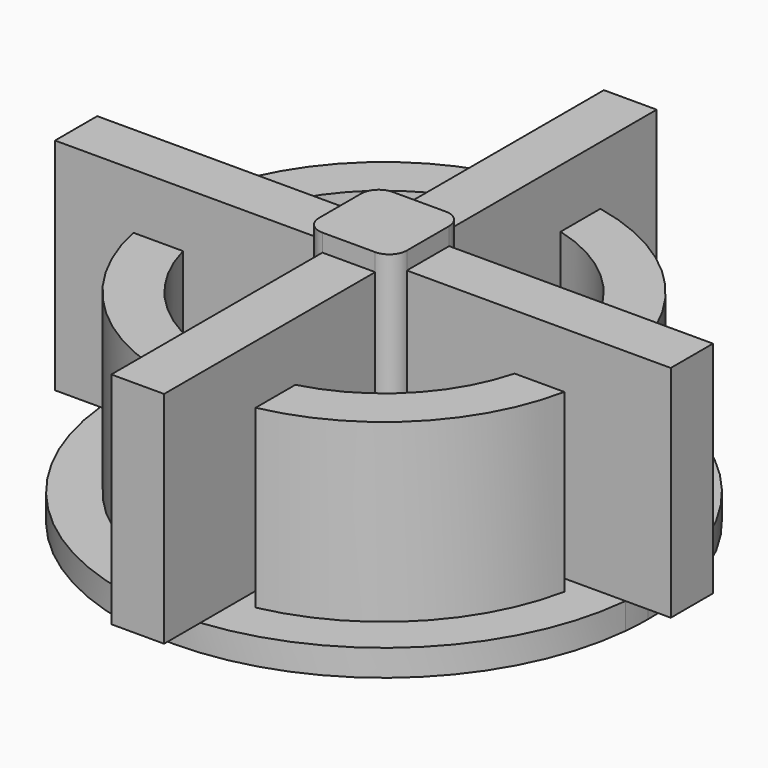
from build123d import *

# Parameters (mm, degrees)
F1_DEPTH = 3
F2_DEPTH = 20
F3_DEPTH = 25
F4_DEPTH = 27


with BuildPart() as f1:
    # F0 (on Top) → F1 (new body)
    with BuildSketch(Plane.XY):
        with BuildLine():
            Line((29.8496231132, -3), (24.819347292, -3))
            ThreePointArc((24.819347292, -3), (24.6773921449, -4.0032882645), (24.4948974278, -5))
            ThreePointArc((24.4948974278, -5), (17.6776695297, -17.6776695297), (5, -24.4948974278))
            ThreePointArc((5, -24.4948974278), (4.0032882645, -24.6773921449), (3, -24.819347292))
            Line((3, -24.819347292), (3, -29.8496231132))
            ThreePointArc((3, -29.8496231132), (21.2132034356, -21.2132034356), (29.8496231132, -3))
        make_face()
        with BuildLine():
            ThreePointArc((5, -24.4948974278), (17.6776695297, -17.6776695297), (24.4948974278, -5))
            Line((24.4948974278, -5), (18.848076825, -5))
            ThreePointArc((18.848076825, -5), (13.7885822331, -13.7885822331), (5, -18.848076825))
            Line((5, -18.848076825), (5, -24.4948974278))
        make_face()
        with BuildLine():
            ThreePointArc((24.4948974278, -5), (24.6773921449, -4.0032882645), (24.819347292, -3))
            Line((24.819347292, -3), (19.267848868, -3))
            ThreePointArc((19.267848868, -3), (19.0841805655, -4.0055027327), (18.848076825, -5))
            Line((18.848076825, -5), (24.4948974278, -5))
        make_face()
        with BuildLine():
            ThreePointArc((25, 0), (24.9547959549, 1.5027171558), (24.819347292, 3))
            Line((24.819347292, 3), (19.267848868, 3))
            ThreePointArc((19.267848868, 3), (19.4418755902, 1.5044844755), (19.5, 0))
            ThreePointArc((19.5, 0), (19.4418755902, -1.5044844755), (19.267848868, -3))
            Line((19.267848868, -3), (24.819347292, -3))
            ThreePointArc((24.819347292, -3), (24.9547959549, -1.5027171558), (25, 0))
        make_face()
        with BuildLine():
            ThreePointArc((24.819347292, 3), (24.6773921449, 4.0032882645), (24.4948974278, 5))
            Line((24.4948974278, 5), (18.848076825, 5))
            ThreePointArc((18.848076825, 5), (19.0841805655, 4.0055027327), (19.267848868, 3))
            Line((19.267848868, 3), (24.819347292, 3))
        make_face()
        with BuildLine():
            Line((18.848076825, 5), (24.4948974278, 5))
            ThreePointArc((24.4948974278, 5), (17.6776695297, 17.6776695297), (5, 24.4948974278))
            Line((5, 24.4948974278), (5, 18.848076825))
            ThreePointArc((5, 18.848076825), (13.7885822331, 13.7885822331), (18.848076825, 5))
        make_face()
        with BuildLine():
            ThreePointArc((5, 24.4948974278), (17.6776695297, 17.6776695297), (24.4948974278, 5))
            ThreePointArc((24.4948974278, 5), (24.6773921449, 4.0032882645), (24.819347292, 3))
            Line((24.819347292, 3), (29.8496231132, 3))
            ThreePointArc((29.8496231132, 3), (21.2132034356, 21.2132034356), (3, 29.8496231132))
            Line((3, 29.8496231132), (3, 24.819347292))
            ThreePointArc((3, 24.819347292), (4.0032882645, 24.6773921449), (5, 24.4948974278))
        make_face()
        with BuildLine():
            Line((29.8496231132, 3), (24.819347292, 3))
            ThreePointArc((24.819347292, 3), (24.9547959549, 1.5027171558), (25, 0))
            ThreePointArc((25, 0), (24.9547959549, -1.5027171558), (24.819347292, -3))
            Line((24.819347292, -3), (29.8496231132, -3))
            ThreePointArc((29.8496231132, -3), (29.9623821933, -1.5018832518), (30, 0))
            ThreePointArc((30, 0), (29.9623821933, 1.5018832518), (29.8496231132, 3))
        make_face()
        with BuildLine():
            ThreePointArc((-3, -29.8496231132), (0, -30), (3, -29.8496231132))
            Line((3, -29.8496231132), (3, -24.819347292))
            ThreePointArc((3, -24.819347292), (0, -25), (-3, -24.819347292))
            Line((-3, -24.819347292), (-3, -29.8496231132))
        make_face()
        with BuildLine():
            ThreePointArc((-3, -24.819347292), (0, -25), (3, -24.819347292))
            Line((3, -24.819347292), (3, -19.267848868))
            ThreePointArc((3, -19.267848868), (0, -19.5), (-3, -19.267848868))
            Line((-3, -19.267848868), (-3, -24.819347292))
        make_face()
        with BuildLine():
            ThreePointArc((3, -24.819347292), (4.0032882645, -24.6773921449), (5, -24.4948974278))
            Line((5, -24.4948974278), (5, -18.848076825))
            ThreePointArc((5, -18.848076825), (4.0055027327, -19.0841805655), (3, -19.267848868))
            Line((3, -19.267848868), (3, -24.819347292))
        make_face()
        with BuildLine():
            ThreePointArc((-5, -24.4948974278), (-4.0032882645, -24.6773921449), (-3, -24.819347292))
            Line((-3, -24.819347292), (-3, -19.267848868))
            ThreePointArc((-3, -19.267848868), (-4.0055027327, -19.0841805655), (-5, -18.848076825))
            Line((-5, -18.848076825), (-5, -24.4948974278))
        make_face()
        with BuildLine():
            Line((-24.819347292, -3), (-29.8496231132, -3))
            ThreePointArc((-29.8496231132, -3), (-21.2132034356, -21.2132034356), (-3, -29.8496231132))
            Line((-3, -29.8496231132), (-3, -24.819347292))
            ThreePointArc((-3, -24.819347292), (-4.0032882645, -24.6773921449), (-5, -24.4948974278))
            ThreePointArc((-5, -24.4948974278), (-17.6776695297, -17.6776695297), (-24.4948974278, -5))
            ThreePointArc((-24.4948974278, -5), (-24.6773921449, -4.0032882645), (-24.819347292, -3))
        make_face()
        with BuildLine():
            Line((-18.848076825, -5), (-24.4948974278, -5))
            ThreePointArc((-24.4948974278, -5), (-17.6776695297, -17.6776695297), (-5, -24.4948974278))
            Line((-5, -24.4948974278), (-5, -18.848076825))
            ThreePointArc((-5, -18.848076825), (-13.7885822331, -13.7885822331), (-18.848076825, -5))
        make_face()
        with BuildLine():
            Line((-19.267848868, -3), (-24.819347292, -3))
            ThreePointArc((-24.819347292, -3), (-24.6773921449, -4.0032882645), (-24.4948974278, -5))
            Line((-24.4948974278, -5), (-18.848076825, -5))
            ThreePointArc((-18.848076825, -5), (-19.0841805655, -4.0055027327), (-19.267848868, -3))
        make_face()
        with BuildLine():
            Line((-19.267848868, 3), (-24.819347292, 3))
            ThreePointArc((-24.819347292, 3), (-25, 0), (-24.819347292, -3))
            Line((-24.819347292, -3), (-19.267848868, -3))
            ThreePointArc((-19.267848868, -3), (-19.5, 0), (-19.267848868, 3))
        make_face()
        with BuildLine():
            Line((-18.848076825, 5), (-24.4948974278, 5))
            ThreePointArc((-24.4948974278, 5), (-24.6773921449, 4.0032882645), (-24.819347292, 3))
            Line((-24.819347292, 3), (-19.267848868, 3))
            ThreePointArc((-19.267848868, 3), (-19.0841805655, 4.0055027327), (-18.848076825, 5))
        make_face()
        with BuildLine():
            ThreePointArc((-5, 24.4948974278), (-4.0032882645, 24.6773921449), (-3, 24.819347292))
            Line((-3, 24.819347292), (-3, 29.8496231132))
            ThreePointArc((-3, 29.8496231132), (-21.2132034356, 21.2132034356), (-29.8496231132, 3))
            Line((-29.8496231132, 3), (-24.819347292, 3))
            ThreePointArc((-24.819347292, 3), (-24.6773921449, 4.0032882645), (-24.4948974278, 5))
            ThreePointArc((-24.4948974278, 5), (-17.6776695297, 17.6776695297), (-5, 24.4948974278))
        make_face()
        with BuildLine():
            Line((-5, 18.848076825), (-5, 24.4948974278))
            ThreePointArc((-5, 24.4948974278), (-17.6776695297, 17.6776695297), (-24.4948974278, 5))
            Line((-24.4948974278, 5), (-18.848076825, 5))
            ThreePointArc((-18.848076825, 5), (-13.7885822331, 13.7885822331), (-5, 18.848076825))
        make_face()
        with BuildLine():
            Line((-3, 19.267848868), (-3, 24.819347292))
            ThreePointArc((-3, 24.819347292), (-4.0032882645, 24.6773921449), (-5, 24.4948974278))
            Line((-5, 24.4948974278), (-5, 18.848076825))
            ThreePointArc((-5, 18.848076825), (-4.0055027327, 19.0841805655), (-3, 19.267848868))
        make_face()
        with BuildLine():
            Line((3, 19.267848868), (3, 24.819347292))
            ThreePointArc((3, 24.819347292), (0, 25), (-3, 24.819347292))
            Line((-3, 24.819347292), (-3, 19.267848868))
            ThreePointArc((-3, 19.267848868), (0, 19.5), (3, 19.267848868))
        make_face()
        with BuildLine():
            Line((5, 18.848076825), (5, 24.4948974278))
            ThreePointArc((5, 24.4948974278), (4.0032882645, 24.6773921449), (3, 24.819347292))
            Line((3, 24.819347292), (3, 19.267848868))
            ThreePointArc((3, 19.267848868), (4.0055027327, 19.0841805655), (5, 18.848076825))
        make_face()
        with BuildLine():
            ThreePointArc((-3, 24.819347292), (0, 25), (3, 24.819347292))
            Line((3, 24.819347292), (3, 29.8496231132))
            ThreePointArc((3, 29.8496231132), (0, 30), (-3, 29.8496231132))
            Line((-3, 29.8496231132), (-3, 24.819347292))
        make_face()
        with BuildLine():
            Line((-24.819347292, 3), (-29.8496231132, 3))
            ThreePointArc((-29.8496231132, 3), (-30, 0), (-29.8496231132, -3))
            Line((-29.8496231132, -3), (-24.819347292, -3))
            ThreePointArc((-24.819347292, -3), (-25, 0), (-24.819347292, 3))
        make_face()
        with BuildLine():
            Line((3, -19.267848868), (3, -5))
            Line((3, -5), (-3, -5))
            Line((-3, -5), (-3, -19.267848868))
            ThreePointArc((-3, -19.267848868), (0, -19.5), (3, -19.267848868))
        make_face()
        with BuildLine():
            ThreePointArc((19.5, 0), (19.4418755902, 1.5044844755), (19.267848868, 3))
            Line((19.267848868, 3), (5, 3))
            Line((5, 3), (5, -3))
            Line((5, -3), (19.267848868, -3))
            ThreePointArc((19.267848868, -3), (19.4418755902, -1.5044844755), (19.5, 0))
        make_face()
        with BuildLine():
            Line((3, 5), (3, 19.267848868))
            ThreePointArc((3, 19.267848868), (0, 19.5), (-3, 19.267848868))
            Line((-3, 19.267848868), (-3, 5))
            Line((-3, 5), (3, 5))
        make_face()
        with BuildLine():
            Line((-5, -3), (-5, 3))
            Line((-5, 3), (-19.267848868, 3))
            ThreePointArc((-19.267848868, 3), (-19.5, 0), (-19.267848868, -3))
            Line((-19.267848868, -3), (-5, -3))
        make_face()
        with BuildLine():
            Line((5, -3), (5, 3))
            ThreePointArc((5, 3), (4.4142135624, 4.4142135624), (3, 5))
            Line((3, 5), (-3, 5))
            ThreePointArc((-3, 5), (-4.4142135624, 4.4142135624), (-5, 3))
            Line((-5, 3), (-5, -3))
            ThreePointArc((-5, -3), (-4.4142135624, -4.4142135624), (-3, -5))
            Line((-3, -5), (3, -5))
            ThreePointArc((3, -5), (4.4142135624, -4.4142135624), (5, -3))
        make_face()
    extrude(amount=-F1_DEPTH)

    # F0 (on Top) → F2 (join)
    with BuildSketch(Plane.XY):
        with BuildLine():
            Line((-5, 18.848076825), (-5, 24.4948974278))
            ThreePointArc((-5, 24.4948974278), (-17.6776695297, 17.6776695297), (-24.4948974278, 5))
            Line((-24.4948974278, 5), (-18.848076825, 5))
            ThreePointArc((-18.848076825, 5), (-13.7885822331, 13.7885822331), (-5, 18.848076825))
        make_face()
        with BuildLine():
            Line((18.848076825, 5), (24.4948974278, 5))
            ThreePointArc((24.4948974278, 5), (17.6776695297, 17.6776695297), (5, 24.4948974278))
            Line((5, 24.4948974278), (5, 18.848076825))
            ThreePointArc((5, 18.848076825), (13.7885822331, 13.7885822331), (18.848076825, 5))
        make_face()
        with BuildLine():
            ThreePointArc((5, -24.4948974278), (17.6776695297, -17.6776695297), (24.4948974278, -5))
            Line((24.4948974278, -5), (18.848076825, -5))
            ThreePointArc((18.848076825, -5), (13.7885822331, -13.7885822331), (5, -18.848076825))
            Line((5, -18.848076825), (5, -24.4948974278))
        make_face()
        with BuildLine():
            Line((-18.848076825, -5), (-24.4948974278, -5))
            ThreePointArc((-24.4948974278, -5), (-17.6776695297, -17.6776695297), (-5, -24.4948974278))
            Line((-5, -24.4948974278), (-5, -18.848076825))
            ThreePointArc((-5, -18.848076825), (-13.7885822331, -13.7885822331), (-18.848076825, -5))
        make_face()
    extrude(amount=F2_DEPTH)

    # F0 (on Top) → F3 (join)
    with BuildSketch(Plane.XY):
        with BuildLine():
            Line((-5, -3), (-5, 3))
            Line((-5, 3), (-19.267848868, 3))
            ThreePointArc((-19.267848868, 3), (-19.5, 0), (-19.267848868, -3))
            Line((-19.267848868, -3), (-5, -3))
        make_face()
        with BuildLine():
            Line((-19.267848868, 3), (-24.819347292, 3))
            ThreePointArc((-24.819347292, 3), (-25, 0), (-24.819347292, -3))
            Line((-24.819347292, -3), (-19.267848868, -3))
            ThreePointArc((-19.267848868, -3), (-19.5, 0), (-19.267848868, 3))
        make_face()
        with BuildLine():
            Line((-24.819347292, 3), (-29.8496231132, 3))
            ThreePointArc((-29.8496231132, 3), (-30, 0), (-29.8496231132, -3))
            Line((-29.8496231132, -3), (-24.819347292, -3))
            ThreePointArc((-24.819347292, -3), (-25, 0), (-24.819347292, 3))
        make_face()
        with BuildLine():
            ThreePointArc((-29.8496231132, -3), (-30, 0), (-29.8496231132, 3))
            Line((-29.8496231132, 3), (-35, 3))
            Line((-35, 3), (-35, -3))
            Line((-35, -3), (-29.8496231132, -3))
        make_face()
        with BuildLine():
            Line((3, -35), (3, -29.8496231132))
            ThreePointArc((3, -29.8496231132), (0, -30), (-3, -29.8496231132))
            Line((-3, -29.8496231132), (-3, -35))
            Line((-3, -35), (3, -35))
        make_face()
        with BuildLine():
            ThreePointArc((-3, -29.8496231132), (0, -30), (3, -29.8496231132))
            Line((3, -29.8496231132), (3, -24.819347292))
            ThreePointArc((3, -24.819347292), (0, -25), (-3, -24.819347292))
            Line((-3, -24.819347292), (-3, -29.8496231132))
        make_face()
        with BuildLine():
            ThreePointArc((-3, -24.819347292), (0, -25), (3, -24.819347292))
            Line((3, -24.819347292), (3, -19.267848868))
            ThreePointArc((3, -19.267848868), (0, -19.5), (-3, -19.267848868))
            Line((-3, -19.267848868), (-3, -24.819347292))
        make_face()
        with BuildLine():
            Line((3, -19.267848868), (3, -5))
            Line((3, -5), (-3, -5))
            Line((-3, -5), (-3, -19.267848868))
            ThreePointArc((-3, -19.267848868), (0, -19.5), (3, -19.267848868))
        make_face()
        with BuildLine():
            ThreePointArc((19.5, 0), (19.4418755902, 1.5044844755), (19.267848868, 3))
            Line((19.267848868, 3), (5, 3))
            Line((5, 3), (5, -3))
            Line((5, -3), (19.267848868, -3))
            ThreePointArc((19.267848868, -3), (19.4418755902, -1.5044844755), (19.5, 0))
        make_face()
        with BuildLine():
            ThreePointArc((25, 0), (24.9547959549, 1.5027171558), (24.819347292, 3))
            Line((24.819347292, 3), (19.267848868, 3))
            ThreePointArc((19.267848868, 3), (19.4418755902, 1.5044844755), (19.5, 0))
            ThreePointArc((19.5, 0), (19.4418755902, -1.5044844755), (19.267848868, -3))
            Line((19.267848868, -3), (24.819347292, -3))
            ThreePointArc((24.819347292, -3), (24.9547959549, -1.5027171558), (25, 0))
        make_face()
        with BuildLine():
            Line((29.8496231132, 3), (24.819347292, 3))
            ThreePointArc((24.819347292, 3), (24.9547959549, 1.5027171558), (25, 0))
            ThreePointArc((25, 0), (24.9547959549, -1.5027171558), (24.819347292, -3))
            Line((24.819347292, -3), (29.8496231132, -3))
            ThreePointArc((29.8496231132, -3), (29.9623821933, -1.5018832518), (30, 0))
            ThreePointArc((30, 0), (29.9623821933, 1.5018832518), (29.8496231132, 3))
        make_face()
        with BuildLine():
            Line((35, 3), (29.8496231132, 3))
            ThreePointArc((29.8496231132, 3), (29.9623821933, 1.5018832518), (30, 0))
            ThreePointArc((30, 0), (29.9623821933, -1.5018832518), (29.8496231132, -3))
            Line((29.8496231132, -3), (35, -3))
            Line((35, -3), (35, 3))
        make_face()
        with BuildLine():
            Line((3, 5), (3, 19.267848868))
            ThreePointArc((3, 19.267848868), (0, 19.5), (-3, 19.267848868))
            Line((-3, 19.267848868), (-3, 5))
            Line((-3, 5), (3, 5))
        make_face()
        with BuildLine():
            Line((3, 19.267848868), (3, 24.819347292))
            ThreePointArc((3, 24.819347292), (0, 25), (-3, 24.819347292))
            Line((-3, 24.819347292), (-3, 19.267848868))
            ThreePointArc((-3, 19.267848868), (0, 19.5), (3, 19.267848868))
        make_face()
        with BuildLine():
            ThreePointArc((-3, 24.819347292), (0, 25), (3, 24.819347292))
            Line((3, 24.819347292), (3, 29.8496231132))
            ThreePointArc((3, 29.8496231132), (0, 30), (-3, 29.8496231132))
            Line((-3, 29.8496231132), (-3, 24.819347292))
        make_face()
        with BuildLine():
            ThreePointArc((-3, 29.8496231132), (0, 30), (3, 29.8496231132))
            Line((3, 29.8496231132), (3, 35))
            Line((3, 35), (-3, 35))
            Line((-3, 35), (-3, 29.8496231132))
        make_face()
    extrude(amount=F3_DEPTH)

    # F0 (on Top) → F4 (join)
    with BuildSketch(Plane.XY):
        with BuildLine():
            Line((5, -3), (5, 3))
            ThreePointArc((5, 3), (4.4142135624, 4.4142135624), (3, 5))
            Line((3, 5), (-3, 5))
            ThreePointArc((-3, 5), (-4.4142135624, 4.4142135624), (-5, 3))
            Line((-5, 3), (-5, -3))
            ThreePointArc((-5, -3), (-4.4142135624, -4.4142135624), (-3, -5))
            Line((-3, -5), (3, -5))
            ThreePointArc((3, -5), (4.4142135624, -4.4142135624), (5, -3))
        make_face()
    extrude(amount=F4_DEPTH)


solid = f1.part
